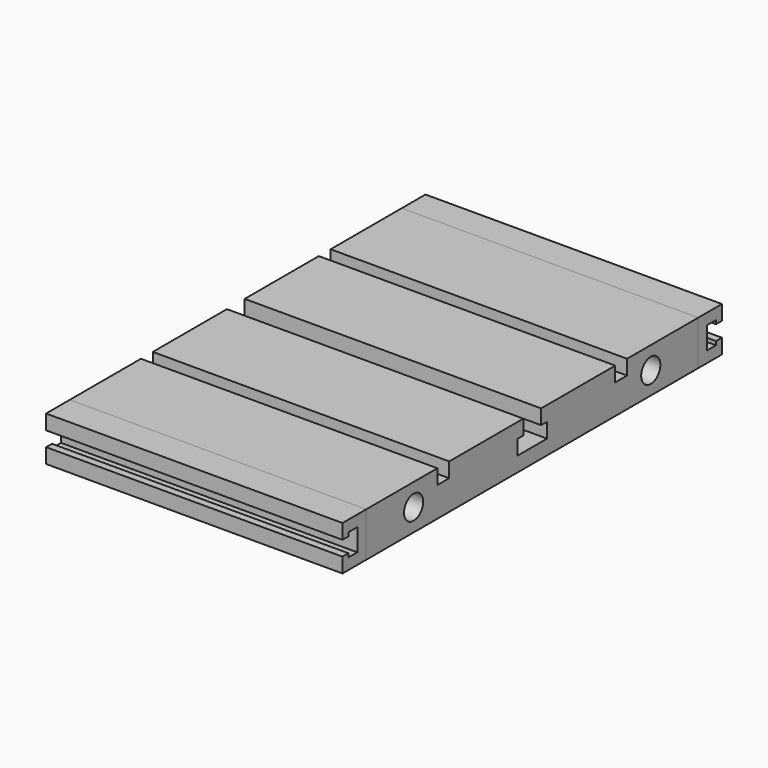
from build123d import *

# Parameters (mm, degrees)
F0_W     = 127
F0_H     = 177.8
F1_DEPTH = 19.05
F2_W     = 6.35
F2_H     = 6.35
F2_W_2   = 9.525
F2_R     = 5.1314415813
F3_DEPTH = 127.001
F5_DEPTH = 127


# Not quite as in the source:
# - a feature names something its author has since deleted; it is built from what else it names


with BuildPart() as f1:
    # F0 (on Top) → F1 (new body)
    with BuildSketch(Plane.XY):
        with Locations((63.5, 88.9)):
            Rectangle(F0_W, F0_H)
    extrude(amount=F1_DEPTH)

    # F2 (on face) → F3 (cut, through all)
    with BuildSketch(Plane.YZ.offset(127)):
        with Locations((41.275, 15.875)):
            Rectangle(F2_W, F2_H)
        with Locations((88.9, 15.875)):
            Rectangle(F2_W_2, F2_H)
        Polygon((93.6625, 12.7), (84.1375, 12.7), (80.9625, 12.7), (80.9625, 6.35), (96.8375, 6.35), (96.8375, 12.7), align=None)
        with Locations((25.4, 9.525)):
            Circle(F2_R)
        with Locations((152.4, 9.525)):
            Circle(F2_R)
        with Locations((136.525, 15.875)):
            Rectangle(F2_W, F2_H)
    extrude(amount=-F3_DEPTH, mode=Mode.SUBTRACT)


with BuildPart() as f5:
    # F4 (on face) → F5 (new body, through all)
    with BuildSketch(Plane.YZ.offset(127)):
        Polygon((0, 0), (0, 19.05), (-12.7, 19.05), (-12.7, 12.7), (-9.525, 12.7), (-9.525, 14.2875), (-4.7625, 14.2875), (-4.7625, 4.7625), (-9.525, 4.7625), (-9.525, 6.35), (-12.7, 6.35), (-12.7, 0), align=None)
    extrude(amount=-F5_DEPTH)


with BuildPart() as f5b:
    # F4 (on face) → F5, piece 2 (new body, through all)
    with BuildSketch(Plane.YZ.offset(127)):
        Polygon((177.8, 19.05), (177.8, 0), (190.5, 0), (190.5, 6.35), (187.325, 6.35), (187.325, 4.7625), (182.5625, 4.7625), (182.5625, 14.2875), (187.325, 14.2875), (187.325, 12.7), (190.5, 12.7), (190.5, 19.05), align=None)
    extrude(amount=-F5_DEPTH)


solid = Compound([f1.part, f5.part, f5b.part])
